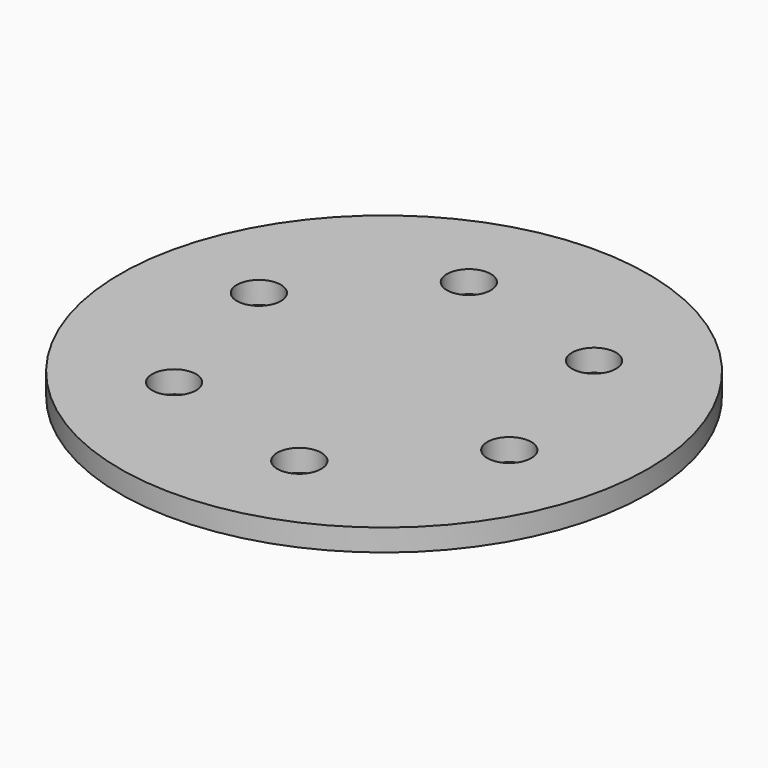
from build123d import *

# Parameters (mm, degrees)
F0_R            = 60
F1_DEPTH        = 5
F3_D            = 10
F3_COPIES_COUNT = 6


# Not quite as in the source:
# - a pattern or mirror of a feature is missing from the dataset's text; its kind, count and spacing are read off the source's solid


with BuildPart() as f1:
    # F0 (on Top) → F1 (new body)
    with BuildSketch(Plane.XY):
        Circle(F0_R)
    extrude(amount=F1_DEPTH)

    # F3 (through all)
    with Locations(Plane.XY.offset(5)):
        with Locations((26.5165042945, 26.5165042945)):
            f3 = Hole(F3_D / 2)

    # F3_copies: F3 ×6 about axis
    f3_copies_axis = Axis((0, 0, 0), (0, 0, 1))
    for i in range(1, F3_COPIES_COUNT):
        add(f3.rotate(f3_copies_axis, i * 360 / F3_COPIES_COUNT), mode=Mode.SUBTRACT)


solid = f1.part
